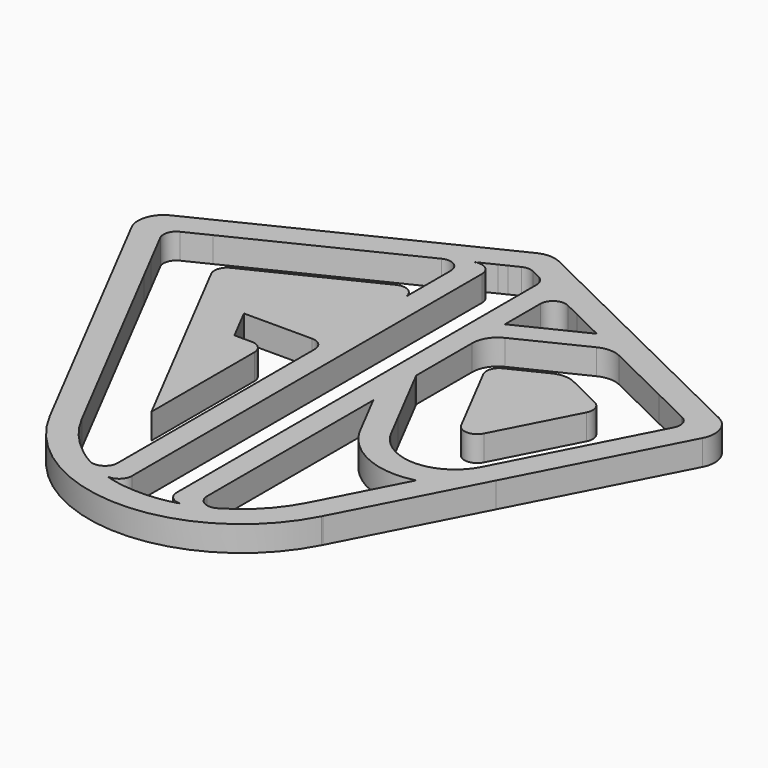
from build123d import *

# Parameters (mm, degrees)
F1_DEPTH = 1


# Not quite as in the source:
# - a feature names something its author has since deleted; it is built from what else it names


with BuildPart() as f1:
    # F0 (on Top) → F1 (new body)
    with BuildSketch(Plane.XY):
        with BuildLine():
            ThreePointArc((-11.7378467649, 8.9264858588), (-12.17732, 9.0282301738), (-12.6167932351, 8.9264858588))
            Line((-12.6167932351, 8.9264858588), (-22.9360292278, 3.8777807945))
            ThreePointArc((-22.9360292278, 3.8777807945), (-23.4460487393, 3.2933140895), (-23.3847383062, 2.5200338931))
            Line((-23.3847383062, 2.5200338931), (-17.5064138811, -8.8425854586))
            ThreePointArc((-17.5064138811, -8.8425854586), (-12.17732, -12.0856381601), (-6.8482261189, -8.8425854586))
            Line((-6.8482261189, -8.8425854586), (-6.8193229677, -8.786716561))
            Line((-6.8193229677, -8.786716561), (-4.1547760271, -3.6362297146))
            Line((-4.1547760271, -3.6362297146), (-0.9699016938, 2.5200338931))
            ThreePointArc((-0.9699016938, 2.5200338931), (-0.9085912607, 3.2933140895), (-1.4186107722, 3.8777807945))
            Line((-1.4186107722, 3.8777807945), (-11.7378467649, 8.9264858588))
        make_face()
        with BuildLine():
            ThreePointArc((-13.9352129405, -9.9781848161), (-14.1856518225, -10.4114506102), (-14.6860899339, -10.4106900001))
            ThreePointArc((-14.6860899339, -10.4106900001), (-14.9764347702, -10.2286994079), (-15.253632646, -10.0272495698))
            ThreePointArc((-15.253632646, -10.0272495698), (-16.0247836651, -9.2789159973), (-16.6182315676, -8.3830942422))
            Line((-16.6182315676, -8.3830942422), (-21.0987998739, 0.2777057515))
            Line((-21.0987998739, 0.2777057515), (-21.5773427489, 1.202714332))
            Line((-21.5773427489, 1.202714332), (-22.2616031934, 2.5253686134))
            ThreePointArc((-22.2616031934, 2.5253686134), (-22.29225841, 2.9120087116), (-22.0372486542, 3.2042420641))
            Line((-22.0372486542, 3.2042420641), (-21.0987998739, 3.6633798445))
            Line((-21.0987998739, 3.6633798445), (-14.6549495581, 6.8160453855))
            ThreePointArc((-14.6549495581, 6.8160453855), (-14.1705134022, 6.7911040048), (-13.9352129405, 6.366917543))
            Line((-13.9352129405, 6.366917543), (-13.9352129405, 4.1403800065))
            ThreePointArc((-13.9352129405, 4.1403800065), (-14.1705134022, 4.5645664683), (-14.6549495581, 4.589507849))
            Line((-14.6549495581, 4.589507849), (-15.253632646, 4.2966010544))
            Line((-15.253632646, 4.2966010544), (-18.9906600384, 2.4682535744))
            Line((-18.9906600384, 2.4682535744), (-18.5866887981, 1.687389658))
            Line((-18.5866887981, 1.687389658), (-16.9010777379, 2.5120779491))
            Line((-16.9010777379, 2.5120779491), (-14.6549495581, 3.6110002651))
            ThreePointArc((-14.6549495581, 3.6110002651), (-14.1705134022, 3.5860588844), (-13.9352129405, 3.1618724226))
            Line((-13.9352129405, 3.1618724226), (-13.9352129405, 1.0737917123))
            Line((-13.9352129405, 1.0737917123), (-13.9352129405, -0.3051582877))
            Line((-13.9352129405, -0.3051582877), (-13.9352129405, -9.9781848161))
        make_face(mode=Mode.SUBTRACT)
        with BuildLine():
            Line((-10.6659804544, -10.8341303593), (-10.4194270595, -10.7664300173))
            ThreePointArc((-10.4194270595, -10.7664300173), (-10.5663720437, -10.8190139832), (-10.7148866004, -10.8669861449))
            ThreePointArc((-10.7148866004, -10.8669861449), (-11.0045154737, -10.9461452883), (-11.2983735297, -11.0077772381))
            ThreePointArc((-11.2983735297, -11.0077772381), (-11.423285282, -11.0284543254), (-11.548680536, -11.0459619827))
            ThreePointArc((-11.548680536, -11.0459619827), (-11.6318465406, -11.0842260567), (-11.720595012, -11.1066856319))
            ThreePointArc((-11.720595012, -11.1066856319), (-12.17732, -11.1424265632), (-12.634044988, -11.1066856319))
            ThreePointArc((-12.634044988, -11.1066856319), (-12.7227934594, -11.0842260567), (-12.805959464, -11.0459619827))
            ThreePointArc((-12.805959464, -11.0459619827), (-12.931354718, -11.0284543254), (-13.0562664703, -11.0077772381))
            ThreePointArc((-13.0562664703, -11.0077772381), (-13.3501245263, -10.9461452883), (-13.6397533997, -10.8669861449))
            ThreePointArc((-13.6397533997, -10.8669861449), (-13.2335773511, -10.7559370641), (-13.0562664703, -10.3740054834))
            Line((-13.0562664703, -10.3740054834), (-13.0562664703, -10.0437429667))
            Line((-13.0562664703, -10.0437429667), (-13.0562664703, 5.3716664708))
            Line((-13.0562664703, 5.3716664708), (-13.0562664703, 6.7969437096))
            ThreePointArc((-13.0562664703, 6.7969437096), (-13.2915669319, 7.2211301714), (-13.7760030878, 7.246071552))
            Line((-13.7760030878, 7.246071552), (-13.0562664703, 7.5982040073))
            Line((-13.0562664703, 7.5982040073), (-12.7760030878, 7.7353233792))
            Line((-12.7760030878, 7.7353233792), (-12.3970566176, 7.9207236322))
            ThreePointArc((-12.3970566176, 7.9207236322), (-12.17732, 7.9715957897), (-11.9575833824, 7.9207236322))
            Line((-11.9575833824, 7.9207236322), (-11.5786369122, 7.7353233792))
            ThreePointArc((-11.5786369122, 7.7353233792), (-11.3741870679, 7.5508950751), (-11.2983735297, 7.2861955367))
            Line((-11.2983735297, 7.2861955367), (-11.2983735297, -10.0437429667))
            Line((-11.2983735297, -10.0437429667), (-11.2983735297, -10.3519767804))
            ThreePointArc((-11.2983735297, -10.3519767804), (-11.1015265128, -10.7495925105), (-10.6659804544, -10.8341303593))
        make_face(mode=Mode.SUBTRACT)
        with BuildLine():
            Line((-5.5053601225, -4.0705468447), (-6.0704119356, -5.1627745276))
            Line((-6.0704119356, -5.1627745276), (-6.8376335928, -6.6457902679))
            Line((-6.8376335928, -6.6457902679), (-7.7364084324, -8.3830942422))
            ThreePointArc((-7.7364084324, -8.3830942422), (-8.5576094615, -9.5349418025), (-9.6685500661, -10.4106900001))
            ThreePointArc((-9.6685500661, -10.4106900001), (-10.1689881775, -10.4114506102), (-10.4194270595, -9.9781848161))
            Line((-10.4194270595, -9.9781848161), (-10.4194270595, -1.8278266693))
            Line((-10.4194270595, -1.8278266693), (-10.4194270595, -0.3051582877))
            Line((-10.4194270595, -0.3051582877), (-10.4194270595, 0.2777057515))
            Line((-10.4194270595, 0.2777057515), (-10.4194270595, 0.5210568374))
            Line((-10.4194270595, 0.5210568374), (-10.4194270595, 3.0275448634))
            Line((-10.4194270595, 3.0275448634), (-10.4194270595, 4.6300693884))
            Line((-10.4194270595, 4.6300693884), (-10.4194270595, 6.366917543))
            Line((-10.4194270595, 6.366917543), (-10.4194270595, 7.1681778407))
            Line((-10.4194270595, 7.1681778407), (-9.6996904419, 6.8160453855))
            Line((-9.6996904419, 6.8160453855), (-9.101007354, 6.5231385909))
            Line((-9.101007354, 6.5231385909), (-7.825559943, 5.8991236145))
            Line((-7.825559943, 5.8991236145), (-6.386082692, 5.1948567393))
            Line((-6.386082692, 5.1948567393), (-3.816366891, 3.9376185884))
            Line((-3.816366891, 3.9376185884), (-2.3768901261, 3.2333519511))
            Line((-2.3768901261, 3.2333519511), (-2.3173913458, 3.2042420641))
            ThreePointArc((-2.3173913458, 3.2042420641), (-2.06238159, 2.9120087116), (-2.0930368066, 2.5253686134))
            Line((-2.0930368066, 2.5253686134), (-2.3768901261, 1.9766889238))
            Line((-2.3768901261, 1.9766889238), (-2.7772972511, 1.202714332))
            Line((-2.7772972511, 1.202714332), (-3.2558401261, 0.2777057515))
            Line((-3.2558401261, 0.2777057515), (-3.3676578126, 0.061565621))
            Line((-3.3676578126, 0.061565621), (-5.0612689658, -3.2121323703))
            Line((-5.0612689658, -3.2121323703), (-5.5053601225, -4.0705468447))
        make_face(mode=Mode.SUBTRACT)
        with BuildLine():
            Line((-16.5720523514, -4.1197169088), (-15.2536327446, -6.6681812422))
            Line((-15.2536327446, -6.6681812422), (-15.2536328928, -1.623578273))
            ThreePointArc((-15.2536328928, -1.623578273), (-15.4000795074, -1.2700248919), (-15.7536328928, -1.1235782877))
            Line((-15.7536328928, -1.1235782877), (-16.0720525039, -1.1235782877))
            Line((-16.0720525039, -1.1235782877), (-16.4336040792, -1.1235782877))
            Line((-16.4336040792, -1.1235782877), (-17.1154396337, 0.1948417123))
            Line((-17.1154396337, 0.1948417123), (-16.0720524345, 0.1948417123))
            Line((-16.0720524345, 0.1948417123), (-15.2536329075, 0.1948417123))
            Line((-15.2536329075, 0.1948417123), (-14.4352129405, 0.1948417123))
            ThreePointArc((-14.4352129405, 0.1948417123), (-14.08165955, 0.0483951029), (-13.9352129405, -0.3051582877))
            Line((-13.9352129405, -0.3051582877), (-13.9352129405, 1.0737917123))
            Line((-13.9352129405, 1.0737917123), (-15.2536329075, 1.0737917123))
            Line((-15.2536329075, 1.0737917123), (-18.2692507427, 1.0737917123))
            Line((-18.2692507427, 1.0737917123), (-18.6097401643, 1.0737917123))
            Line((-18.6097401643, 1.0737917123), (-19.1218068604, 0.8088797168))
            Line((-19.1218068604, 0.8088797168), (-16.5720523514, -4.1197169088))
        make_face()
        Polygon((-16.1325828631, -3.0563212317), (-16.6777508926, -2.0025282877), (-16.1325828631, -2.0025282877), (-16.1325828631, -2.6348403451), align=None, mode=Mode.SUBTRACT)
        with BuildLine():
            Line((-15.2536329075, 1.0737917123), (-13.9352129405, 1.0737917123))
            Line((-13.9352129405, 1.0737917123), (-13.9352129405, 3.1618724226))
            ThreePointArc((-13.9352129405, 3.1618724226), (-14.1705134022, 3.5860588844), (-14.6549495581, 3.6110002651))
            Line((-14.6549495581, 3.6110002651), (-16.9010777379, 2.5120779491))
            Line((-16.9010777379, 2.5120779491), (-18.5866887981, 1.687389658))
            Line((-18.5866887981, 1.687389658), (-18.3411390159, 1.2127495215))
            Line((-18.3411390159, 1.2127495215), (-18.2692507427, 1.0737917123))
            Line((-18.2692507427, 1.0737917123), (-15.2536329075, 1.0737917123))
        make_face()
        with BuildLine():
            ThreePointArc((-9.101007354, -4.2055538888), (-7.7228805899, -5.1184524182), (-6.0704119356, -5.1627745276))
            Line((-6.0704119356, -5.1627745276), (-5.5053601225, -4.0705468447))
            Line((-5.5053601225, -4.0705468447), (-5.0612689658, -3.2121323703))
            ThreePointArc((-5.0612689658, -3.2121323703), (-6.8376335928, -4.2931499375), (-8.6139982198, -3.2121323703))
            Line((-8.6139982198, -3.2121323703), (-9.101007354, -2.2707587726))
            Line((-9.101007354, -2.2707587726), (-9.101007354, -4.2055538888))
        make_face()
        with BuildLine():
            Line((-10.4194270595, 4.6300693884), (-10.4194270595, 3.0275448634))
            ThreePointArc((-10.4194270595, 3.0275448634), (-10.2677999831, 3.5569439401), (-9.8589002946, 3.9258005484))
            Line((-9.8589002946, 3.9258005484), (-7.2650291622, 5.1948567393))
            ThreePointArc((-7.2650291622, 5.1948567393), (-6.8255559271, 5.2966010544), (-6.386082692, 5.1948567393))
            Line((-6.386082692, 5.1948567393), (-7.825559943, 5.8991236145))
            Line((-7.825559943, 5.8991236145), (-9.7711979643, 4.9472166576))
            Line((-9.7711979643, 4.9472166576), (-10.4194270595, 4.6300693884))
        make_face()
        with BuildLine():
            ThreePointArc((-9.4838699082, -3.6362297146), (-9.3087674014, -3.9318726716), (-9.101007354, -4.2055538888))
            Line((-9.101007354, -4.2055538888), (-9.101007354, -2.2707587726))
            Line((-9.101007354, -2.2707587726), (-10.307609373, 0.061565621))
            Line((-10.307609373, 0.061565621), (-10.4194270595, 0.2777057515))
            Line((-10.4194270595, 0.2777057515), (-10.4194270595, -0.3051582877))
            Line((-10.4194270595, -0.3051582877), (-10.4194270595, -1.8278266693))
            Line((-10.4194270595, -1.8278266693), (-9.4838699082, -3.6362297146))
        make_face()
        with BuildLine():
            Line((-19.5454273692, 1.6277250617), (-19.3764089282, 1.3010176414))
            Line((-19.3764089282, 1.3010176414), (-18.5866887981, 1.687389658))
            Line((-18.5866887981, 1.687389658), (-18.9906600384, 2.4682535744))
            Line((-18.9906600384, 2.4682535744), (-19.32107283, 2.3065985124))
            ThreePointArc((-19.32107283, 2.3065985124), (-19.5760825858, 2.01436516), (-19.5454273692, 1.6277250617))
        make_face()
        Polygon((-19.3764089282, 1.3010176414), (-19.1218068604, 0.8088797168), (-18.6097401643, 1.0737917123), (-18.3411390159, 1.2127495215), (-18.5866887981, 1.687389658), align=None)
        Polygon((-16.1325828631, -2.0025282877), (-16.6777508926, -2.0025282877), (-16.1325828631, -3.0563212317), (-16.1325828631, -2.6348403451), align=None)
        with BuildLine():
            Line((-10.4194270595, 7.1681778407), (-10.4194270595, 6.366917543))
            ThreePointArc((-10.4194270595, 6.366917543), (-10.1841265978, 6.7911040048), (-9.6996904419, 6.8160453855))
            Line((-9.6996904419, 6.8160453855), (-10.4194270595, 7.1681778407))
        make_face()
        with BuildLine():
            ThreePointArc((-11.720595012, -11.1066856319), (-11.6318465406, -11.0842260567), (-11.548680536, -11.0459619827))
            ThreePointArc((-11.548680536, -11.0459619827), (-12.17732, -11.0856381601), (-12.805959464, -11.0459619827))
            ThreePointArc((-12.805959464, -11.0459619827), (-12.7227934594, -11.0842260567), (-12.634044988, -11.1066856319))
            ThreePointArc((-12.634044988, -11.1066856319), (-12.17732, -11.1424265632), (-11.720595012, -11.1066856319))
        make_face()
        Polygon((-18.3411390159, 1.2127495215), (-18.6097401643, 1.0737917123), (-18.2692507427, 1.0737917123), align=None)
        with BuildLine():
            ThreePointArc((-10.7148866004, -10.8669861449), (-10.5663720437, -10.8190139832), (-10.4194270595, -10.7664300173))
            Line((-10.4194270595, -10.7664300173), (-10.6659804544, -10.8341303593))
            ThreePointArc((-10.6659804544, -10.8341303593), (-11.1015265128, -10.7495925105), (-11.2983735297, -10.3519767804))
            Line((-11.2983735297, -10.3519767804), (-11.2983735297, -10.3740054834))
            ThreePointArc((-11.2983735297, -10.3740054834), (-11.1210626489, -10.7559370641), (-10.7148866004, -10.8669861449))
        make_face()
    extrude(amount=F1_DEPTH)


with BuildPart() as f1b:
    # F0 (on Top) → F1, piece 2 (new body)
    with BuildSketch(Plane.XY):
        with BuildLine():
            ThreePointArc((-7.2817247495, -1.4347354631), (-6.8376335928, -1.7049898549), (-6.393542436, -1.4347354631))
            Line((-6.393542436, -1.4347354631), (-4.8092126308, 1.6277250617))
            ThreePointArc((-4.8092126308, 1.6277250617), (-4.7785574142, 2.01436516), (-5.03356717, 2.3065985124))
            Line((-5.03356717, 2.3065985124), (-6.3981603577, 2.9742282228))
            ThreePointArc((-6.3981603577, 2.9742282228), (-6.6120850226, 3.0502044622), (-6.8376335928, 3.0759725378))
            ThreePointArc((-6.8376335928, 3.0759725378), (-7.063182163, 3.0502044622), (-7.2771068279, 2.9742282228))
            Line((-7.2771068279, 2.9742282228), (-8.6417000156, 2.3065985124))
            ThreePointArc((-8.6417000156, 2.3065985124), (-8.8967097713, 2.01436516), (-8.8660545548, 1.6277250617))
            Line((-8.8660545548, 1.6277250617), (-7.2817247495, -1.4347354631))
        make_face()
        Polygon((-6.8581561948, 2.2207744428), (-6.8376335928, 2.2107337222), (-5.7679512019, 1.687389658), (-6.8376335928, -0.3802733283), (-7.9034853086, 1.6799850815), align=None, mode=Mode.SUBTRACT)
        Polygon((-5.7679512019, 1.687389658), (-6.8376335928, 2.2107337222), (-6.8581561948, 2.2207744428), (-7.9034853086, 1.6799850815), (-6.8376335928, -0.3802733283), align=None)
    extrude(amount=F1_DEPTH)


solid = Compound([f1.part, f1b.part])
